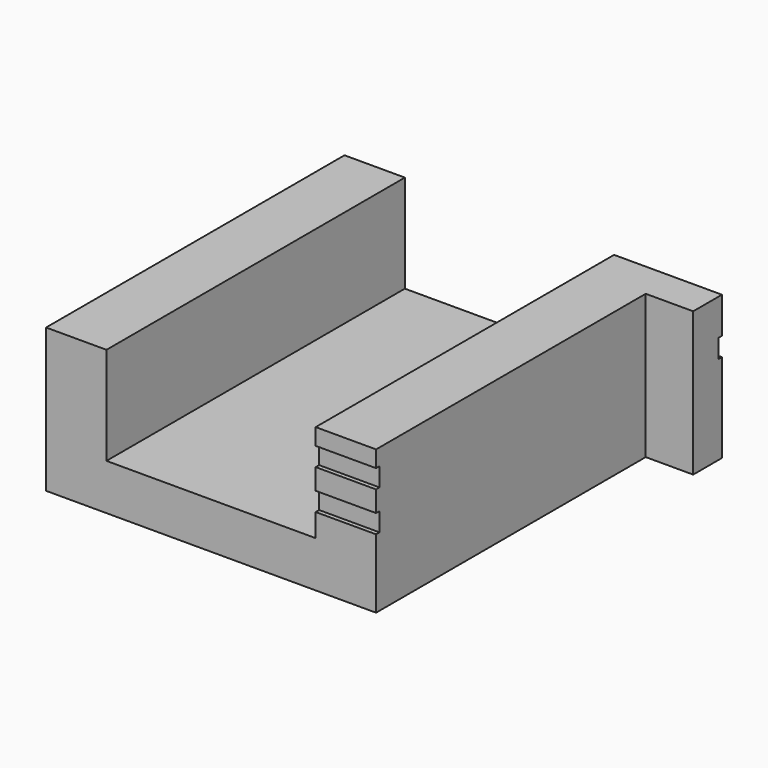
from build123d import *

# Parameters (mm, degrees)
F1_DEPTH = 8.128
F0_W     = 10.668
F0_H     = 65.8876
F0_W_2   = 8.382
F0_H_2   = 6.35
F2_DEPTH = 25.4
F3_W     = 10.668
F3_H     = 3.302
F4_DEPTH = 0.762
F5_W     = 19.05
F5_H     = 3.302
F6_DEPTH = 0.762


# Not quite as in the source:
# - a feature names something its author has since deleted; it is built from what else it names


with BuildPart() as f1:
    # F0 (on Top) → F1 (new body)
    with BuildSketch(Plane.XY):
        Polygon((18.4785, -32.9438), (18.4785, 32.9438), (-1.905, 32.9438), (-18.4785, 32.9438), (-18.4785, -32.9438), (-9.652, -32.9438), (9.652, -32.9438), align=None)
    extrude(amount=F1_DEPTH)

    # F0 (on Top) → F2 (join)
    with BuildSketch(Plane.XY):
        with Locations((-23.8125, 0)):
            Rectangle(F0_W, F0_H)
        with Locations((33.3375, 29.7688)):
            Rectangle(F0_W_2, F0_H_2)
        Polygon((29.1465, 26.5938), (29.1465, 32.9438), (18.4785, 32.9438), (18.4785, -32.9438), (29.1465, -32.9438), (29.1465, -20.2438), align=None)
    extrude(amount=F2_DEPTH)

    # F3 (on face) → F4 (cut)
    with BuildSketch(Plane.XZ.offset(32.9438)):
        with Locations((23.8125, 13.843)):
            Rectangle(F3_W, F3_H)
        with Locations((23.8125, 20.828)):
            Rectangle(F3_W, F3_H)
    extrude(amount=-F4_DEPTH, mode=Mode.SUBTRACT)

    # F5 (on face) → F6 (cut)
    with BuildSketch(Plane(origin=(0, 32.9438, 0), x_dir=(-1, 0, 0), z_dir=(0, 1, 0))):
        with Locations((-28.0035, 17.3482)):
            Rectangle(F5_W, F5_H)
    extrude(amount=-F6_DEPTH, mode=Mode.SUBTRACT)


solid = f1.part
